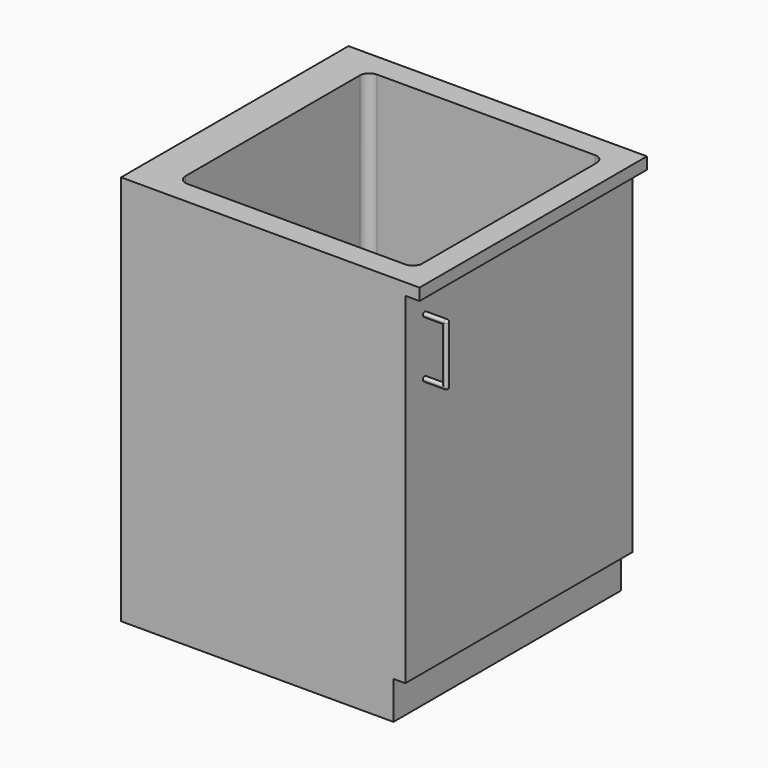
from build123d import *

# Parameters (mm, degrees)
F0_W        = 600
F0_H        = 600
F1_DEPTH    = 800
F2_W        = 600
F2_H        = 80
F3_DEPTH    = 25
F5_DEPTH    = 50
F6_T1_DEPTH = 120
F6_T4_ANGLE = 180
F6_T6_ANGLE = 180
F7_W        = 40
F7_H        = 110
F8_DEPTH    = 25
F9_R        = 4.99999
F10_W       = 630
F10_H       = 600
F11_DEPTH   = 25
F13_DEPTH   = 400
F14_R       = 5
F16_D       = 50
F16_DEPTH   = 40
F16_TIP     = 15.0215154757


# Not quite as in the source:
# - a fillet or chamfer that OpenCascade refuses, or shapes differently, is made with other operations: its cross-section is extruded or revolved along the edge and cut away or added
# - a fillet or chamfer is up to 0.001 mm smaller than in the source, because OpenCascade refuses the exact size


with BuildPart() as f1:
    # F0 (on Top) → F1 (new body)
    with BuildSketch(Plane.XY):
        Rectangle(F0_W, F0_H)
    extrude(amount=F1_DEPTH)

    # F2 (on face) → F3 (cut)
    with BuildSketch(Plane.YZ.offset(300)):
        with Locations((0, 40)):
            Rectangle(F2_W, F2_H)
    extrude(amount=-F3_DEPTH, mode=Mode.SUBTRACT)

    # F4 (on face) → F5 (join)
    with BuildSketch(Plane.YZ.offset(300)):
        with BuildLine():
            ThreePointArc((-248.5795542598, 750), (-252.1150881657, 748.5355339059), (-253.5795542598, 745))
            Line((-253.5795542598, 745), (-253.5795542598, 625))
            ThreePointArc((-253.5795542598, 625), (-252.1150881657, 621.4644660941), (-248.5795542598, 620))
            ThreePointArc((-248.5795542598, 620), (-245.0440203538, 621.4644660941), (-243.5795542598, 625))
            Line((-243.5795542598, 625), (-243.5795542598, 745))
            ThreePointArc((-243.5795542598, 745), (-245.0440203538, 748.5355339059), (-248.5795542598, 750))
        make_face()
    extrude(amount=F5_DEPTH)

    # F6: fillet of radius 5 on 4 edges, made by hand

    # F6_s2 → F6_t1 (cut)
    with BuildSketch(Plane.XY.offset(625)):
        with BuildLine():
            ThreePointArc((345, -253.5795542598), (348.5355339059, -252.1150881657), (350, -248.5795542598))
            Line((350, -248.5795542598), (350, -253.5795542598))
            Line((350, -253.5795542598), (345, -253.5795542598))
        make_face()
        with BuildLine():
            ThreePointArc((345, -243.5795542598), (348.5355339059, -245.0440203538), (350, -248.5795542598))
            Line((350, -248.5795542598), (350, -243.5795542598))
            Line((350, -243.5795542598), (345, -243.5795542598))
        make_face()
    extrude(amount=F6_T1_DEPTH, mode=Mode.SUBTRACT)

    # F6_s3 → F6_t4 (revolve, cut)
    with BuildSketch(Plane.XY.offset(745)):
        with BuildLine():
            ThreePointArc((345, -253.5795542598), (348.5355339059, -252.1150881657), (350, -248.5795542598))
            Line((350, -248.5795542598), (350, -253.5795542598))
            Line((350, -253.5795542598), (345, -253.5795542598))
        make_face()
    revolve(axis=Axis((350, -248.5795542598, 745), (-1, 0, 0)), revolution_arc=F6_T4_ANGLE, mode=Mode.SUBTRACT)

    # F6_s5 → F6_t6 (revolve, cut)
    with BuildSketch(Plane.XY.offset(625)):
        with BuildLine():
            ThreePointArc((345, -243.5795542598), (348.5355339059, -245.0440203538), (350, -248.5795542598))
            Line((350, -248.5795542598), (350, -243.5795542598))
            Line((350, -243.5795542598), (345, -243.5795542598))
        make_face()
    revolve(axis=Axis((350, -248.5795542598, 625), (-1, 0, 0)), revolution_arc=F6_T6_ANGLE, mode=Mode.SUBTRACT)

    # F7 (on face) → F8 (cut)
    with BuildSketch(Plane(origin=(0, -243.5795542598, 0), x_dir=(-1, 0, 0), z_dir=(0, 1, 0))):
        with Locations((-320, 685)):
            Rectangle(F7_W, F7_H)
    extrude(amount=-F8_DEPTH, mode=Mode.SUBTRACT)

    # F9 (radius 5 in the source; OpenCascade refuses exactly that, so slightly less here)
    f9_edges = [f1.edges().sort_by_distance(p)[0] for p in [
        (320, -243.579554, 740),
        (340, -243.579554, 685),
        (320, -243.579554, 630),
        (320, -253.579554, 740),
        (340, -253.579554, 685),
        (320, -253.579554, 630),
    ]]
    fillet(f9_edges, radius=F9_R)

    # F10 (on face) → F11 (join)
    with BuildSketch(Plane.XY.offset(800)):
        with Locations((15, 0)):
            Rectangle(F10_W, F10_H)
    extrude(amount=F11_DEPTH)

    # F12 (on face) → F13 (cut)
    with BuildSketch(Plane.XY.offset(825)):
        with BuildLine():
            Line((-200, -250), (260, -250))
            ThreePointArc((260, -250), (274.1421356237, -244.1421356237), (280, -230))
            Line((280, -230), (280, 230))
            ThreePointArc((280, 230), (274.1421356237, 244.1421356237), (260, 250))
            Line((260, 250), (-200, 250))
            ThreePointArc((-200, 250), (-214.1421356237, 244.1421356237), (-220, 230))
            Line((-220, 230), (-220, -230))
            ThreePointArc((-220, -230), (-214.1421356237, -244.1421356237), (-200, -250))
        make_face()
    extrude(amount=-F13_DEPTH, mode=Mode.SUBTRACT)

    # F14
    f14_edges = [f1.edges().sort_by_distance(p)[0] for p in [
        (30, 250, 425),
        (-214.142136, 244.142136, 425),
        (-220, 0, 425),
        (30, -250, 425),
        (274.142136, -244.142136, 425),
        (280, 0, 425),
        (274.142136, 244.142136, 425),
        (-214.142136, -244.142136, 425),
    ]]
    fillet(f14_edges, radius=F14_R)

    # F16
    with Locations(Plane.XY.offset(425)):
        with Locations((-127.0953565836, 0)):
            Hole(F16_D / 2, depth=F16_DEPTH)
            with Locations((0, 0, -(F16_DEPTH + F16_TIP / 2))):  # 118° drill point
                Cone(0, F16_D / 2, F16_TIP, mode=Mode.SUBTRACT)


solid = f1.part
